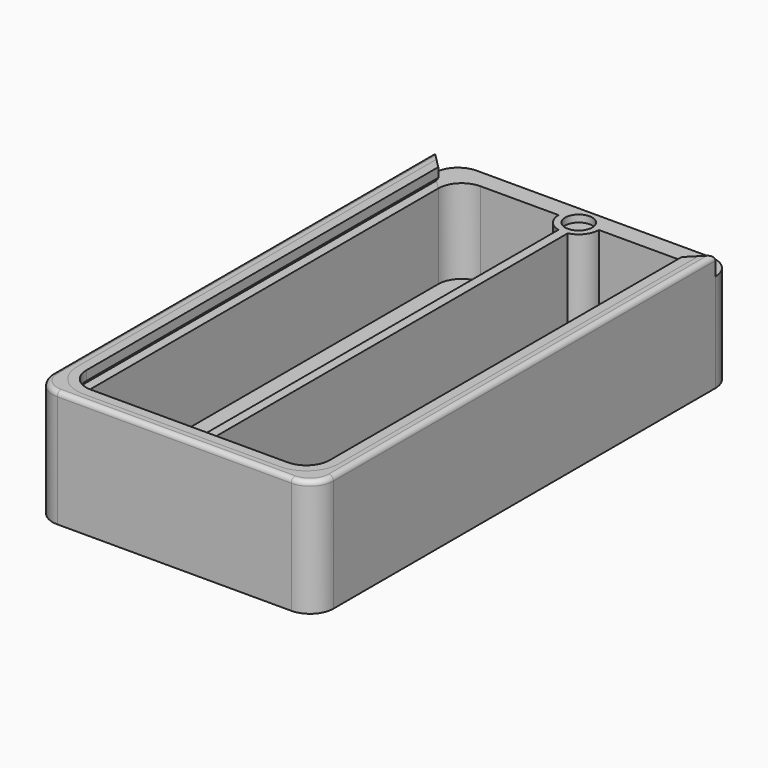
from build123d import *

# Parameters (mm, degrees)
F0_R     = 2.9
F1_DEPTH = 21
F2_DEPTH = 3
F3_DEPTH = 19.5
F4_DEPTH = 25
F5_DEPTH = 25
F6_W     = 150
F6_H     = 2
F7_DEPTH = 35
F8_DEPTH = 2
F9_SIZE  = 1.99999
F10_R    = 1


# Not quite as in the source:
# - a fillet or chamfer is up to 0.001 mm smaller than in the source, because OpenCascade refuses the exact size
# - a feature names something its author has since deleted; it is built from what else it names


with BuildPart() as f1:
    # F0 (on Top) → F1 (new body)
    with BuildSketch(Plane.XY):
        with BuildLine():
            Line((28.249738031, 48.17828843), (4.8277114148, 48.17828843))
            ThreePointArc((4.8277114148, 48.17828843), (6.8046842718, 46.5974530016), (7.549738031, 44.17828843))
            Line((7.549738031, 44.17828843), (24.249738031, 44.17828843))
            ThreePointArc((24.249738031, 44.17828843), (27.7852719369, 42.7138223359), (29.249738031, 39.17828843))
            Line((29.249738031, 39.17828843), (31.249738031, 41.17828843))
            Line((31.249738031, 41.17828843), (33.249738031, 43.17828843))
            ThreePointArc((33.249738031, 43.17828843), (31.7852719369, 46.7138223359), (28.249738031, 48.17828843))
        make_face()
        with BuildLine():
            Line((1.6717646472, 48.17828843), (-21.750261969, 48.17828843))
            ThreePointArc((-21.750261969, 48.17828843), (-25.285795875, 46.7138223359), (-26.750261969, 43.17828843))
            Line((-26.750261969, 43.17828843), (-24.750261969, 41.17828843))
            Line((-24.750261969, 41.17828843), (-22.750261969, 39.17828843))
            ThreePointArc((-22.750261969, 39.17828843), (-21.285795875, 42.7138223359), (-17.750261969, 44.17828843))
            Line((-17.750261969, 44.17828843), (-1.050261969, 44.17828843))
            ThreePointArc((-1.050261969, 44.17828843), (-0.3052082099, 46.5974530016), (1.6717646472, 48.17828843))
        make_face()
        with BuildLine():
            ThreePointArc((4.249738031, 39.9961836967), (3.249738031, 39.87828843), (2.249738031, 39.9961836967))
            Line((2.249738031, 39.9961836967), (2.249738031, -56.82171157))
            ThreePointArc((2.249738031, -56.82171157), (1.3710583745, -58.9430319136), (-0.750261969, -59.82171157))
            Line((-0.750261969, -59.82171157), (7.249738031, -59.82171157))
            ThreePointArc((7.249738031, -59.82171157), (5.1284176874, -58.9430319136), (4.249738031, -56.82171157))
            Line((4.249738031, -56.82171157), (4.249738031, 39.9961836967))
        make_face()
        with BuildLine():
            Line((4.8277114148, 48.17828843), (1.6717646472, 48.17828843))
            ThreePointArc((1.6717646472, 48.17828843), (-0.3052082099, 46.5974530016), (-1.050261969, 44.17828843))
            ThreePointArc((-1.050261969, 44.17828843), (-0.125910055, 41.5146443096), (2.249738031, 39.9961836967))
            ThreePointArc((2.249738031, 39.9961836967), (3.249738031, 39.87828843), (4.249738031, 39.9961836967))
            ThreePointArc((4.249738031, 39.9961836967), (6.6253861169, 41.5146443096), (7.549738031, 44.17828843))
            ThreePointArc((7.549738031, 44.17828843), (6.8046842718, 46.5974530016), (4.8277114148, 48.17828843))
        make_face()
        with Locations((3.249738031, 44.17828843)):
            Circle(F0_R, mode=Mode.SUBTRACT)
    extrude(amount=F1_DEPTH)

    # F0 (on Top) → F2 (join)
    with BuildSketch(Plane.XY):
        with BuildLine():
            ThreePointArc((2.249738031, 39.9961836967), (-0.125910055, 41.5146443096), (-1.050261969, 44.17828843))
            Line((-1.050261969, 44.17828843), (-17.750261969, 44.17828843))
            ThreePointArc((-17.750261969, 44.17828843), (-21.285795875, 42.7138223359), (-22.750261969, 39.17828843))
            Line((-22.750261969, 39.17828843), (-22.750261969, -54.82171157))
            ThreePointArc((-22.750261969, -54.82171157), (-21.285795875, -58.357245476), (-17.750261969, -59.82171157))
            Line((-17.750261969, -59.82171157), (-0.750261969, -59.82171157))
            ThreePointArc((-0.750261969, -59.82171157), (1.3710583745, -58.9430319136), (2.249738031, -56.82171157))
            Line((2.249738031, -56.82171157), (2.249738031, 39.9961836967))
        make_face()
        with BuildLine():
            Line((24.249738031, 44.17828843), (7.549738031, 44.17828843))
            ThreePointArc((7.549738031, 44.17828843), (6.6253861169, 41.5146443096), (4.249738031, 39.9961836967))
            Line((4.249738031, 39.9961836967), (4.249738031, -56.82171157))
            ThreePointArc((4.249738031, -56.82171157), (5.1284176874, -58.9430319136), (7.249738031, -59.82171157))
            Line((7.249738031, -59.82171157), (24.249738031, -59.82171157))
            ThreePointArc((24.249738031, -59.82171157), (27.7852719369, -58.357245476), (29.249738031, -54.82171157))
            Line((29.249738031, -54.82171157), (29.249738031, 39.17828843))
            ThreePointArc((29.249738031, 39.17828843), (27.7852719369, 42.7138223359), (24.249738031, 44.17828843))
        make_face()
    extrude(amount=F2_DEPTH)

    # F0 (on Top) → F3 (join)
    with BuildSketch(Plane.XY):
        with BuildLine():
            Line((-24.750261969, 41.17828843), (-26.750261969, 43.17828843))
            Line((-26.750261969, 43.17828843), (-26.750261969, -58.82171157))
            ThreePointArc((-26.750261969, -58.82171157), (-25.285795875, -62.357245476), (-21.750261969, -63.82171157))
            Line((-21.750261969, -63.82171157), (28.249738031, -63.82171157))
            ThreePointArc((28.249738031, -63.82171157), (31.7852719369, -62.357245476), (33.249738031, -58.82171157))
            Line((33.249738031, -58.82171157), (33.249738031, 43.17828843))
            Line((33.249738031, 43.17828843), (31.249738031, 41.17828843))
            Line((31.249738031, 41.17828843), (31.249738031, -54.82171157))
            ThreePointArc((31.249738031, -54.82171157), (29.1994854993, -59.7714590383), (24.249738031, -61.82171157))
            Line((24.249738031, -61.82171157), (-17.750261969, -61.82171157))
            ThreePointArc((-17.750261969, -61.82171157), (-22.7000094373, -59.7714590383), (-24.750261969, -54.82171157))
            Line((-24.750261969, -54.82171157), (-24.750261969, 41.17828843))
        make_face()
        with Locations((3.249738031, 44.17828843)):
            Circle(F0_R)
    extrude(amount=F3_DEPTH)

    # F0 (on Top) → F4 (join)
    with BuildSketch(Plane.XY):
        with BuildLine():
            Line((-24.750261969, 41.17828843), (-26.750261969, 43.17828843))
            Line((-26.750261969, 43.17828843), (-26.750261969, -58.82171157))
            ThreePointArc((-26.750261969, -58.82171157), (-25.285795875, -62.357245476), (-21.750261969, -63.82171157))
            Line((-21.750261969, -63.82171157), (28.249738031, -63.82171157))
            ThreePointArc((28.249738031, -63.82171157), (31.7852719369, -62.357245476), (33.249738031, -58.82171157))
            Line((33.249738031, -58.82171157), (33.249738031, 43.17828843))
            Line((33.249738031, 43.17828843), (31.249738031, 41.17828843))
            Line((31.249738031, 41.17828843), (31.249738031, -54.82171157))
            ThreePointArc((31.249738031, -54.82171157), (29.1994854993, -59.7714590383), (24.249738031, -61.82171157))
            Line((24.249738031, -61.82171157), (-17.750261969, -61.82171157))
            ThreePointArc((-17.750261969, -61.82171157), (-22.7000094373, -59.7714590383), (-24.750261969, -54.82171157))
            Line((-24.750261969, -54.82171157), (-24.750261969, 41.17828843))
        make_face()
    extrude(amount=F4_DEPTH)

    # F10
    f10_edges = [f1.edges().sort_by_distance(p)[0] for p in [
        (33.249738, -7.821712, 25),
        (31.785272, -62.357245, 25),
        (-26.750262, -7.821712, 25),
        (-25.285796, -62.357245, 25),
        (3.249738, -63.821712, 25),
    ]]
    fillet(f10_edges, radius=F10_R)


with BuildPart() as f5:
    # F0 (on Top) → F5 (new body)
    with BuildSketch(Plane.XY):
        with BuildLine():
            Line((-22.750261969, 39.17828843), (-24.750261969, 41.17828843))
            Line((-24.750261969, 41.17828843), (-24.750261969, -54.82171157))
            ThreePointArc((-24.750261969, -54.82171157), (-22.7000094373, -59.7714590383), (-17.750261969, -61.82171157))
            Line((-17.750261969, -61.82171157), (24.249738031, -61.82171157))
            ThreePointArc((24.249738031, -61.82171157), (29.1994854993, -59.7714590383), (31.249738031, -54.82171157))
            Line((31.249738031, -54.82171157), (31.249738031, 41.17828843))
            Line((31.249738031, 41.17828843), (29.249738031, 39.17828843))
            Line((29.249738031, 39.17828843), (29.249738031, -54.82171157))
            ThreePointArc((29.249738031, -54.82171157), (27.7852719369, -58.357245476), (24.249738031, -59.82171157))
            Line((24.249738031, -59.82171157), (7.249738031, -59.82171157))
            Line((7.249738031, -59.82171157), (-0.750261969, -59.82171157))
            Line((-0.750261969, -59.82171157), (-17.750261969, -59.82171157))
            ThreePointArc((-17.750261969, -59.82171157), (-21.285795875, -58.357245476), (-22.750261969, -54.82171157))
            Line((-22.750261969, -54.82171157), (-22.750261969, 39.17828843))
        make_face()
    extrude(amount=F5_DEPTH)

    # F6 (on Right) → F7 (cut, symmetric)
    with BuildSketch(Plane.YZ):
        with Locations((-12.0285183191, 22)):
            Rectangle(F6_W, F6_H)
    extrude(amount=F7_DEPTH, both=True, mode=Mode.SUBTRACT)


with BuildPart() as f8:
    # F8 (new): a face of the model
    f8_faces = [f5.part.faces().sort_by_distance(p)[0] for p in [
        (30.4221287508, -7.82171157, 23),
    ]]
    extrude(f8_faces, amount=F8_DEPTH)

    # F9 (size 2 in the source; OpenCascade refuses exactly that, so slightly less here)
    f9_edges = [f8.edges().sort_by_distance(p)[0] for p in [
        (-22.750262, -7.821712, 21),
    ]]
    chamfer(f9_edges, length=F9_SIZE)


solid = Compound([f1.part, f5.part, f8.part])
